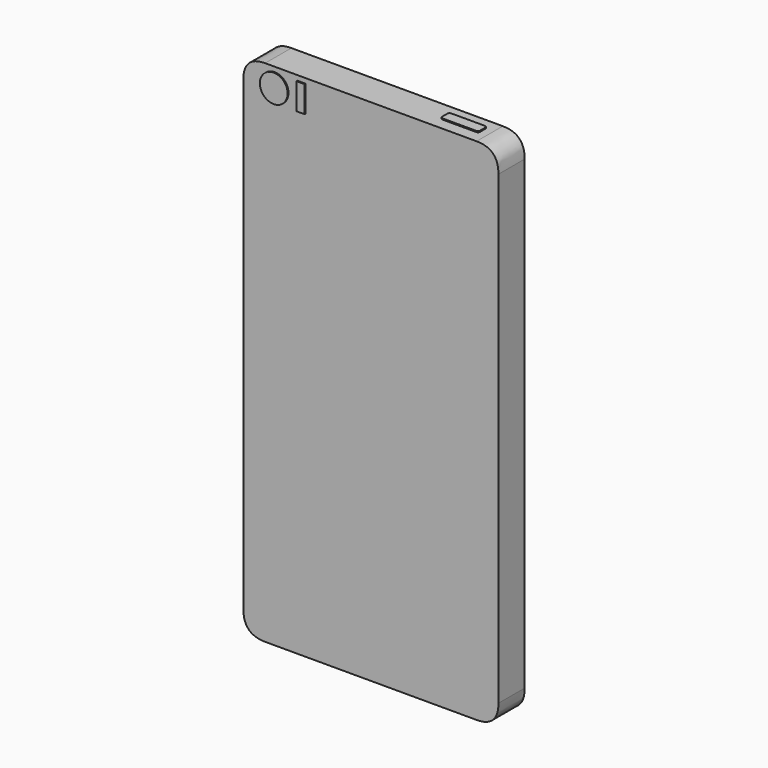
from build123d import *

# Parameters (mm, degrees)
F0_W         = 59.3232400715
F0_H         = 118.4509694576
F1_DEPTH     = 7.62
F2_T1_DEPTH  = 33.02
F3_T1_DEPTH  = 33.02
F4_T1_DEPTH  = 33.02
F5_T1_DEPTH  = 33.02
F17_W        = 8.8130328804
F17_H        = 2.5180093944
F18_DEPTH    = 0.254
F19_T1_DEPTH = 1.524
F20_R        = 0.508
F10_R        = 2.8607169915
F21_DEPTH    = 0.254
F11_R        = 2.8607134233
F22_DEPTH    = 0.254
F12_W        = 1.611137297
F12_H        = 7.3773153126
F23_DEPTH    = 0.254
F7_R         = 1.0781434008
F24_DEPTH    = 0.254
F9_W         = 6.8501718342
F9_H         = 1.6440376639
F25_DEPTH    = 0.254
F13_R        = 3.228368755
F26_DEPTH    = 0.254
F14_W        = 1.9021295011
F14_H        = 6.1539448798
F27_DEPTH    = 0.254
F8_R         = 3.0136808832
F28_DEPTH    = 0.254
F6_W         = 58.911472559
F6_H         = 101.9305512309
F29_DEPTH    = 0.254
F16_W        = 8.6615839973
F16_H        = 2.4723988026
F30_DEPTH    = 0.762
F15_R        = 2.8680658163
F31_DEPTH    = 0.762


# Not quite as in the source:
# - a fillet or chamfer that OpenCascade refuses, or shapes differently, is made with other operations: its cross-section is extruded or revolved along the edge and cut away or added


with BuildPart() as f1:
    # F0 (on Front) → F1 (new body)
    with BuildSketch(Plane.XZ):
        Rectangle(F0_W, F0_H)
    extrude(amount=F1_DEPTH)

    # F2: fillet of radius 5.08 on 1 edges, made by hand

    # F2_s2 → F2_t1 (cut)
    with BuildSketch(Plane.XZ.offset(-12.7)):
        with BuildLine():
            add(Edge.make_bspline(
                [(29.6616200358, 54.1454847288), (29.6616200358, 59.2254847288), (24.5816200358, 59.2254847288)],
                knots=[0, 0, 0, 1, 1, 1], degree=2, weights=[1, 1, 1]))
            Line((24.5816200358, 59.2254847288), (29.6616200358, 59.2254847288))
            Line((29.6616200358, 59.2254847288), (29.6616200358, 54.1454847288))
        make_face()
    extrude(amount=F2_T1_DEPTH, mode=Mode.SUBTRACT)

    # F3: fillet of radius 5.08 on 1 edges, made by hand

    # F3_s2 → F3_t1 (cut)
    with BuildSketch(Plane.XZ.offset(-12.7)):
        with BuildLine():
            add(Edge.make_bspline(
                [(-29.6616200358, 54.1454847288), (-29.6616200358, 59.2254847288), (-24.5816200358, 59.2254847288)],
                knots=[0, 0, 0, 1, 1, 1], degree=2, weights=[1, 1, 1]))
            Line((-24.5816200358, 59.2254847288), (-29.6616200358, 59.2254847288))
            Line((-29.6616200358, 59.2254847288), (-29.6616200358, 54.1454847288))
        make_face()
    extrude(amount=F3_T1_DEPTH, mode=Mode.SUBTRACT)

    # F4: fillet of radius 5.08 on 1 edges, made by hand

    # F4_s2 → F4_t1 (cut)
    with BuildSketch(Plane.XZ.offset(-12.7)):
        with BuildLine():
            add(Edge.make_bspline(
                [(-24.5816200358, -59.2254847288), (-29.6616200358, -59.2254847288), (-29.6616200358, -54.1454847288)],
                knots=[0, 0, 0, 1, 1, 1], degree=2, weights=[1, 1, 1]))
            Line((-29.6616200358, -54.1454847288), (-29.6616200358, -59.2254847288))
            Line((-29.6616200358, -59.2254847288), (-24.5816200358, -59.2254847288))
        make_face()
    extrude(amount=F4_T1_DEPTH, mode=Mode.SUBTRACT)

    # F5: fillet of radius 5.08 on 1 edges, made by hand

    # F5_s2 → F5_t1 (cut)
    with BuildSketch(Plane.XZ.offset(-12.7)):
        with BuildLine():
            add(Edge.make_bspline(
                [(29.6616200358, -54.1454847288), (29.6616200358, -59.2254847288), (24.5816200358, -59.2254847288)],
                knots=[0, 0, 0, 1, 1, 1], degree=2, weights=[1, 1, 1]))
            Line((24.5816200358, -59.2254847288), (29.6616200358, -59.2254847288))
            Line((29.6616200358, -59.2254847288), (29.6616200358, -54.1454847288))
        make_face()
    extrude(amount=F5_T1_DEPTH, mode=Mode.SUBTRACT)

    # F17 (on face) → F18 (join)
    with BuildSketch(Plane.XY.offset(59.2254847288)):
        with Locations((18.3535870165, -3.5715140402)):
            Rectangle(F17_W, F17_H)
    extrude(amount=F18_DEPTH)

    # F19: fillet of radius 0.508 on 1 edges, made by hand

    # F19_s2 → F19_t1 (cut)
    with BuildSketch(Plane.XY.offset(59.2254847288)):
        with BuildLine():
            add(Edge.make_bspline(
                [(22.2521034567, -2.312509343), (22.7601034567, -2.312509343), (22.7601034567, -2.820509343)],
                knots=[0, 0, 0, 1, 1, 1], degree=2, weights=[1, 1, 1]))
            Line((22.7601034567, -2.820509343), (22.7601034567, -2.312509343))
            Line((22.7601034567, -2.312509343), (22.2521034567, -2.312509343))
        make_face()
    extrude(amount=F19_T1_DEPTH, mode=Mode.SUBTRACT)

    # F20
    f20_edges = [f1.edges().sort_by_distance(p)[0] for p in [
        (13.947071, -2.312509, 59.352485),
        (22.760103, -4.830519, 59.352485),
        (13.947071, -4.830519, 59.352485),
    ]]
    fillet(f20_edges, radius=F20_R)

    # F10 (on face) → F21 (join)
    with BuildSketch(Plane(origin=(-29.6616200358, 0, 0), x_dir=(0, -1, 0), z_dir=(-1, 0, 0))):
        with Locations((3.9731003344, 38.3609607816)):
            Circle(F10_R)
    extrude(amount=F21_DEPTH)

    # F11 (on face) → F22 (join)
    with BuildSketch(Plane(origin=(-29.6616200358, 0, 0), x_dir=(0, -1, 0), z_dir=(-1, 0, 0))):
        with Locations((3.9731003344, 28.7707187235)):
            Circle(F11_R)
    extrude(amount=F22_DEPTH)

    # F12 (on face) → F23 (join)
    with BuildSketch(Plane(origin=(-29.6616200358, 0, 0), x_dir=(0, -1, 0), z_dir=(-1, 0, 0))):
        with Locations((3.8694504183, 49.0038786083)):
            Rectangle(F12_W, F12_H)
    extrude(amount=F23_DEPTH)

    # F7 (on face) → F24 (join)
    with BuildSketch(Plane(origin=(0, 0, 0), x_dir=(-1, 0, 0), z_dir=(0, 1, 0))):
        with Locations((0, 56.2707670033)):
            Circle(F7_R)
    extrude(amount=F24_DEPTH)

    # F9 (on face) → F25 (join)
    with BuildSketch(Plane(origin=(0, 0, 0), x_dir=(-1, 0, 0), z_dir=(0, 1, 0))):
        with Locations((0, 53.4313358366)):
            Rectangle(F9_W, F9_H)
    extrude(amount=F25_DEPTH)

    # F13 (on face) → F26 (join)
    with BuildSketch(Plane.XZ.offset(7.62)):
        with Locations((-22.3876349628, 54.8886656761)):
            Circle(F13_R)
    extrude(amount=F26_DEPTH)

    # F14 (on face) → F27 (join)
    with BuildSketch(Plane.XZ.offset(7.62)):
        with Locations((-16.1777436733, 55.0005566329)):
            Rectangle(F14_W, F14_H)
    extrude(amount=F27_DEPTH)

    # F8 (on Front) → F28 (join)
    with BuildSketch(Plane.XZ):
        with Locations((0, -55.3571693599)):
            Circle(F8_R)
    extrude(amount=-F28_DEPTH)

    # F6 (on Front) → F29 (join)
    with BuildSketch(Plane.XZ):
        Rectangle(F6_W, F6_H)
    extrude(amount=-F29_DEPTH)

    # F16 (on face) → F30 (cut)
    with BuildSketch(Plane(origin=(0, 0, -59.2254847288), x_dir=(1, 0, 0), z_dir=(0, 0, -1))):
        with Locations((0, 4.0924949571)):
            Rectangle(F16_W, F16_H)
    extrude(amount=-F30_DEPTH, mode=Mode.SUBTRACT)

    # F15 (on face) → F31 (cut)
    with BuildSketch(Plane(origin=(0, 0, -59.2254847288), x_dir=(1, 0, 0), z_dir=(0, 0, -1))):
        with Locations((19.5690467954, 3.8177834358)):
            Circle(F15_R)
    extrude(amount=-F31_DEPTH, mode=Mode.SUBTRACT)


solid = f1.part
